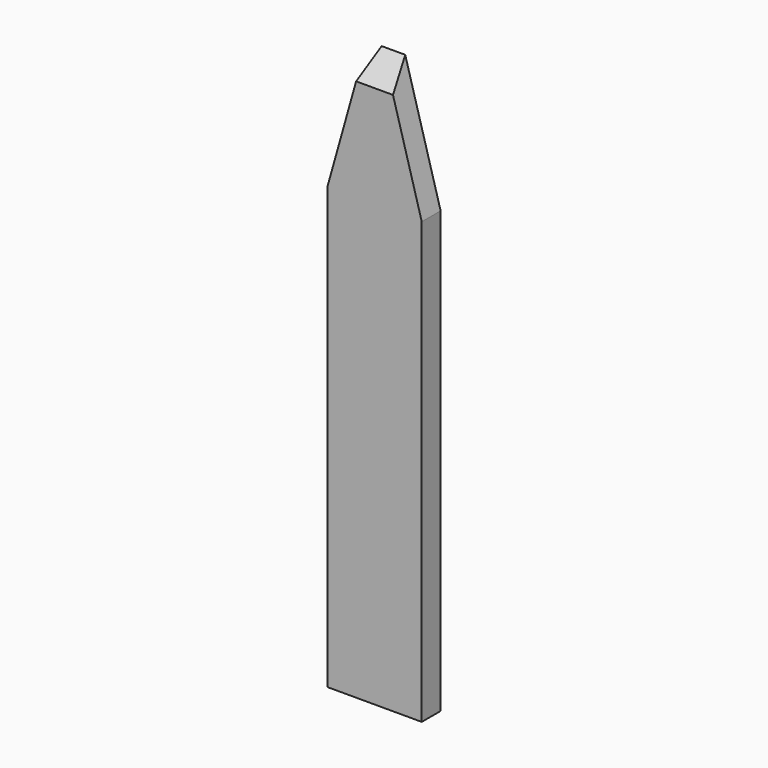
from build123d import *

# Parameters (mm, degrees)
F0_W     = 76.2
F0_H     = 457.2
F1_DEPTH = 19.05
F3_DEPTH = 19.051
F4_SIZE  = 19.04999


# Not quite as in the source:
# - a fillet or chamfer is up to 0.001 mm smaller than in the source, because OpenCascade refuses the exact size


with BuildPart() as f1:
    # F0 (on Front) → F1 (new body)
    with BuildSketch(Plane.XZ):
        with Locations((38.1, 228.6)):
            Rectangle(F0_W, F0_H)
    extrude(amount=F1_DEPTH)

    # F2 (on face) → F3 (cut, through all)
    with BuildSketch(Plane.XZ.offset(19.05)):
        Polygon((0, 355.6), (28.575, 457.2), (0, 457.2), align=None)
        Polygon((76.2, 457.2), (47.625, 457.2), (76.2, 355.6), align=None)
    extrude(amount=-F3_DEPTH, mode=Mode.SUBTRACT)

    # F4 (size 19.05 in the source; OpenCascade refuses exactly that, so slightly less here)
    f4_edges = [f1.edges().sort_by_distance(p)[0] for p in [
        (38.1, -19.05, 457.2),
    ]]
    chamfer(f4_edges, length=F4_SIZE)


solid = f1.part
